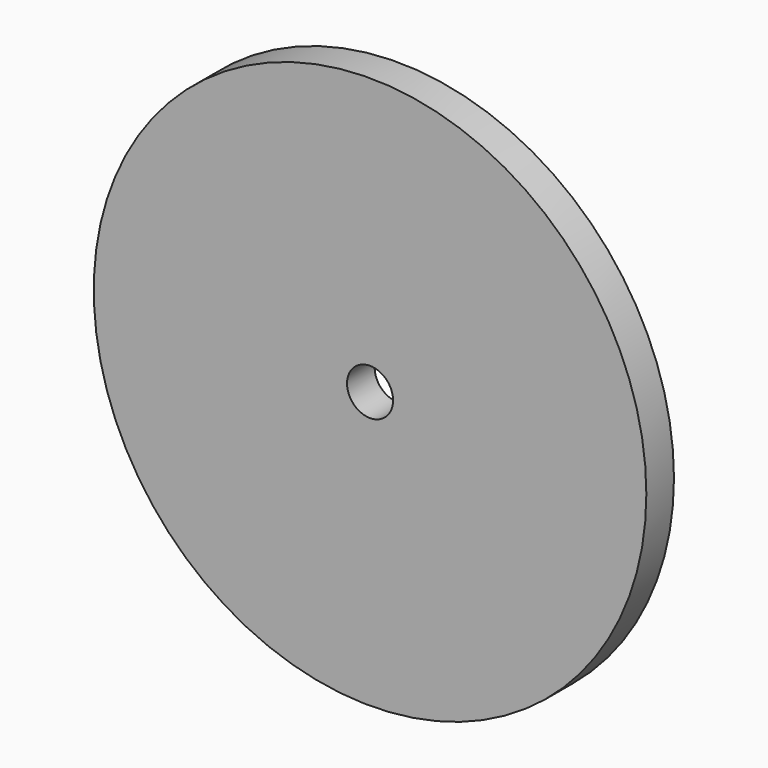
from build123d import *

# Parameters (mm, degrees)
F0_R     = 38.1
F0_R_2   = 3.175
F1_DEPTH = 4.7625


# Not quite as in the source:
# - a length typed as a fraction of an inch, garbled in the dataset ("3 / 203.2 mm" for 3/8 in), is restored


with BuildPart() as f1:
    # F0 (on Front) → F1 (new body)
    with BuildSketch(Plane.XZ):
        Circle(F0_R)
        Circle(F0_R_2, mode=Mode.SUBTRACT)
    extrude(amount=F1_DEPTH)


solid = f1.part
